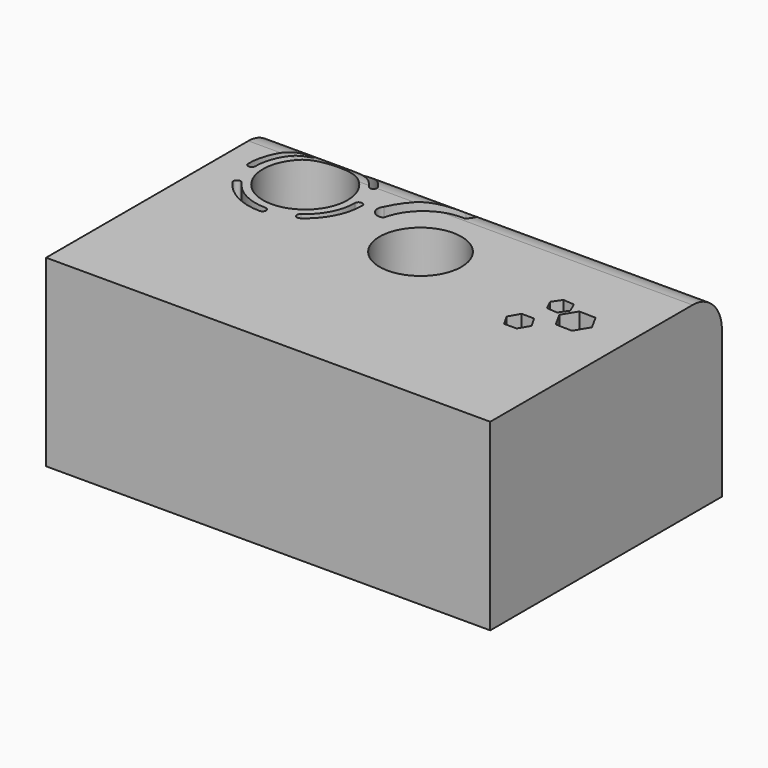
from build123d import *

# Parameters (mm, degrees)
F0_W        = 61.4208132029
F0_H        = 40.0461480021
F0_R        = 5.8356598506
F0_R_2      = 5.6623382773
F1_DEPTH    = 25.4
F2_T1_DEPTH = 86.8208132029


# Not quite as in the source:
# - a fillet or chamfer that OpenCascade refuses, or shapes differently, is made with other operations: its cross-section is extruded or revolved along the edge and cut away or added


with BuildPart() as f1:
    # F0 (on Top) → F1 (new body)
    with BuildSketch(Plane.XY):
        with Locations((9.6422955394, -0.2926178277)):
            Rectangle(F0_W, F0_H)
        with BuildLine():
            ThreePointArc((-15.5581902422, 6.5874267261), (-13.0892777006, 4.4019793182), (-9.8877530545, 3.6133415997))
            ThreePointArc((-9.8877530545, 3.6133415997), (-9.3918088824, 3.1173974276), (-9.8877530545, 2.6214532554))
            ThreePointArc((-9.8877530545, 2.6214532554), (-13.525571131, 3.5108261592), (-16.3427069667, 5.9783046702))
            ThreePointArc((-16.3427069667, 5.9783046702), (-16.2723997648, 6.6975216235), (-15.5581902422, 6.5874267261))
        make_face(mode=Mode.SUBTRACT)
        with BuildLine():
            ThreePointArc((-5.9691235315, 4.8356190614), (-3.7836761236, 7.304531603), (-2.9950384051, 10.5060562491))
            ThreePointArc((-2.9950384051, 10.5060562491), (-2.4990942329, 11.0020004213), (-2.0031500608, 10.5060562491))
            ThreePointArc((-2.0031500608, 10.5060562491), (-2.8925229646, 6.8682381727), (-5.3600014756, 4.051102337))
            ThreePointArc((-5.3600014756, 4.051102337), (-6.0792184289, 4.1214095389), (-5.9691235315, 4.8356190614))
        make_face(mode=Mode.SUBTRACT)
        with BuildLine():
            ThreePointArc((-13.8063825775, 16.1764934369), (-15.9918299854, 13.7075808953), (-16.7804677039, 10.5060562491))
            ThreePointArc((-16.7804677039, 10.5060562491), (-17.2764118761, 10.010112077), (-17.7723560482, 10.5060562491))
            ThreePointArc((-17.7723560482, 10.5060562491), (-16.8829831444, 14.1438743256), (-14.4155046334, 16.9610101613))
            ThreePointArc((-14.4155046334, 16.9610101613), (-13.6962876801, 16.8907029594), (-13.8063825775, 16.1764934369))
        make_face(mode=Mode.SUBTRACT)
        with Locations((-9.8877530545, 10.5060562491)):
            Circle(F0_R, mode=Mode.SUBTRACT)
        with BuildLine():
            ThreePointArc((-9.8877530545, 17.3987708986), (-10.3836972266, 17.8947150707), (-9.8877530545, 18.3906592429))
            ThreePointArc((-9.8877530545, 18.3906592429), (-6.249934978, 17.5012863391), (-3.4327991423, 15.0338078281))
            ThreePointArc((-3.4327991423, 15.0338078281), (-3.5031063442, 14.3145908748), (-4.2173158668, 14.4246857722))
            ThreePointArc((-4.2173158668, 14.4246857722), (-6.6862284084, 16.6101331801), (-9.8877530545, 17.3987708986))
        make_face(mode=Mode.SUBTRACT)
        with BuildLine():
            ThreePointArc((6.6644512117, 17.5767932087), (8.5373270865, 17.0581119265), (8.5140671581, 15.1148792356))
            ThreePointArc((8.5140671581, 15.1148792356), (4.0257871944, 13.7216332626), (1.5243776143, 9.7430981696))
            ThreePointArc((1.5243776143, 9.7430981696), (-0.0147844439, 10.1939229676), (0, 11.7976823822))
            ThreePointArc((0, 11.7976823822), (2.6892272592, 15.4287413311), (6.6644512117, 17.5767932087))
        make_face(mode=Mode.SUBTRACT)
        with Locations((9.6422955394, 6.0194581747)):
            Circle(F0_R_2, mode=Mode.SUBTRACT)
        Polygon((28.9662275463, 1.5064948219), (29.8360027373, 0), (28.9662275463, -1.5064948219), (27.2266771644, -1.5064948219), (26.3569019735, 0), (27.2266771644, 1.5064948219), align=None, mode=Mode.SUBTRACT)
        Polygon((33.9459068477, 1.8158181313), (31.6559560597, 1.8676351756), (30.5558555424, 3.8766992536), (31.7457058131, 5.8339462873), (34.0356566012, 5.782129243), (35.1357571185, 3.773065165), align=None, mode=Mode.SUBTRACT)
        Polygon((30.2401456875, 6.7547236703), (30.8922100812, 5.3890366107), (30.0355225909, 4.141488751), (28.5267707068, 4.259627951), (27.874706313, 5.6253150105), (28.7313938034, 6.8728628702), align=None, mode=Mode.SUBTRACT)
    extrude(amount=F1_DEPTH)

    # F2: fillet of radius 5.08 on 1 edges, made by hand

    # F2_s2 → F2_t1 (cut)
    with BuildSketch(Plane.YZ.offset(-33.768111062)):
        with BuildLine():
            ThreePointArc((19.7304561734, 20.32), (18.2425586218, 23.9121024484), (14.6504561734, 25.4))
            Line((14.6504561734, 25.4), (19.7304561734, 25.4))
            Line((19.7304561734, 25.4), (19.7304561734, 20.32))
        make_face()
    extrude(amount=F2_T1_DEPTH, mode=Mode.SUBTRACT)


solid = f1.part
